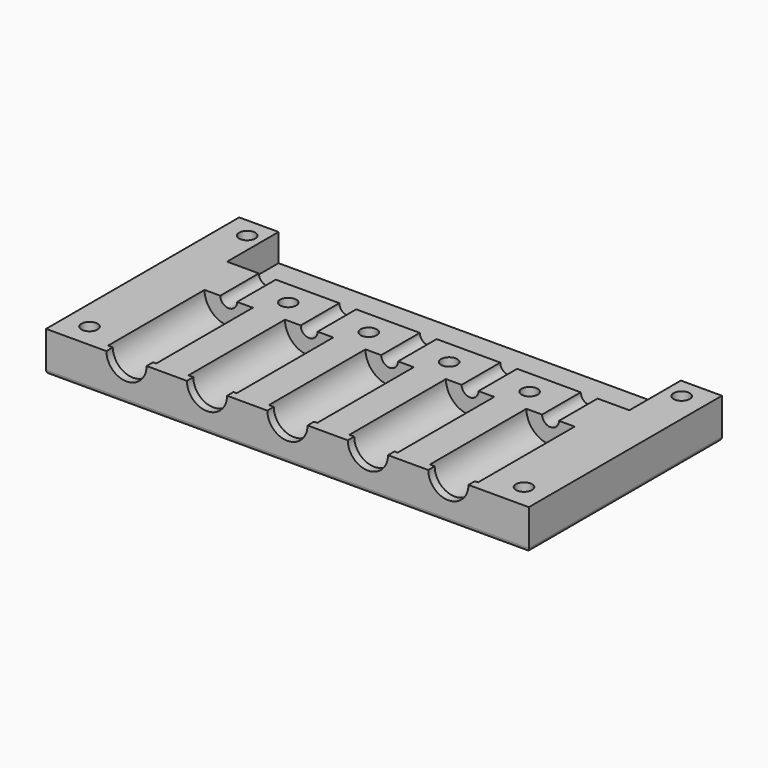
from build123d import *

# Parameters (mm, degrees)
F0_W      = 60
F0_H      = 25
F1_DEPTH  = 5
F2_R      = 2.5
F3_DEPTH  = 10
F5_R      = 3
F6_DEPTH  = 15
F7_R      = 1.05
F8_DEPTH  = 29
F9_W      = 50
F9_H      = 3.4154356362
F10_DEPTH = 3
F11_DEPTH = 5
F12_R     = 0.5
F14_R     = 1
F13_R     = 1
F15_DEPTH = 5.001
F16_R     = 1
F17_DEPTH = 5.001
F18_SIZE  = 1


with BuildPart() as f1:
    # F0 (on Top) → F1 (new body)
    with BuildSketch(Plane.XY):
        with Locations((-2.9453901201, -7.2920476746)):
            Rectangle(F0_W, F0_H)
    extrude(amount=F1_DEPTH)

    # F2 (on face) → F3 (cut)
    with BuildSketch(Plane.XZ.offset(19.7920476746)):
        with Locations((-22.9453901201, 5)):
            Circle(F2_R)
        with Locations((-12.9453901201, 5)):
            Circle(F2_R)
        with Locations((-2.9453901201, 5)):
            Circle(F2_R)
        with Locations((7.0546098799, 5)):
            Circle(F2_R)
        with Locations((17.0546098799, 5)):
            Circle(F2_R)
    extrude(amount=-F3_DEPTH, mode=Mode.SUBTRACT)

    # F5 (on offset) → F6 (cut)
    with BuildSketch(Plane.XZ.offset(18.7920476746)):
        with Locations((-23.0476632714, 5.0127296709)):
            Circle(F5_R)
        with Locations((-13.0476632714, 5.0127296709)):
            Circle(F5_R)
        with Locations((-3.0476632714, 5.0127296709)):
            Circle(F5_R)
        with Locations((6.9523367286, 5.0127296709)):
            Circle(F5_R)
        with Locations((16.9523367286, 5.0127296709)):
            Circle(F5_R)
    extrude(amount=-F6_DEPTH, mode=Mode.SUBTRACT)

    # F7 (on face) → F8 (cut)
    with BuildSketch(Plane.XZ.offset(3.7920476746)):
        with Locations((-23.0476632714, 5.0127296709)):
            Circle(F7_R)
        with Locations((-13.0476632714, 5.0127296709)):
            Circle(F7_R)
        with Locations((-3.0476632714, 5.0127296709)):
            Circle(F7_R)
        with Locations((6.9523367286, 5.0127296709)):
            Circle(F7_R)
        with Locations((16.9523367286, 5.0127296709)):
            Circle(F7_R)
    extrude(amount=-F8_DEPTH, mode=Mode.SUBTRACT)

    # F9 (on face) → F10 (cut)
    with BuildSketch(Plane(origin=(0, 5.2079523254, 0), x_dir=(-1, 0, 0), z_dir=(0, 1, 0))):
        with Locations((3.0476632714, 3.2922821819)):
            Rectangle(F9_W, F9_H)
    extrude(amount=-F10_DEPTH, mode=Mode.SUBTRACT)

    # F11 (add): a face of the model
    f11_faces = [f1.faces().sort_by_distance(p)[0] for p in [
        (-2.8102387692, 5.2079523254, 1.4530193808),
    ]]
    extrude(f11_faces, amount=F11_DEPTH)

    # F12
    f12_edges = [f1.edges().sort_by_distance(p)[0] for p in [
        (27.05461, -4.792048, 0),
        (-2.94539, -19.792048, 0),
        (-32.94539, -4.792048, 0),
    ]]
    fillet(f12_edges, radius=F12_R)

    # F14 (on face) + F13 (on face) → F15 (cut, through all)
    with BuildSketch(Plane(origin=(0, 0, 0), x_dir=(1, 0, 0), z_dir=(0, 0, -1))):
        with Locations((-29.9453901201, -7.7079523254)):
            Circle(F14_R)
        with Locations((24.0546098799, -7.7079523254)):
            Circle(F14_R)
    with BuildSketch(Plane(origin=(0, 0, 0), x_dir=(1, 0, 0), z_dir=(0, 0, -1))):
        with Locations((-29.9453901201, 16.7920476746)):
            Circle(F13_R)
        with Locations((24.0546098799, 16.7920476746)):
            Circle(F13_R)
    extrude(amount=-F15_DEPTH, mode=Mode.SUBTRACT)

    # F16 (on face) → F17 (cut, through all)
    with BuildSketch(Plane.XY.offset(5)):
        with Locations((11.9524138955, -0.7920476746)):
            Circle(F16_R)
        with Locations((1.9524138955, -0.7920476746)):
            Circle(F16_R)
        with Locations((-8.0475861045, -0.7920476746)):
            Circle(F16_R)
        with Locations((-18.0475861045, -0.7920476746)):
            Circle(F16_R)
    extrude(amount=-F17_DEPTH, mode=Mode.SUBTRACT)

    # F18
    f18_edges = [f1.edges().sort_by_distance(p)[0] for p in [
        (23.05461, 7.707952, 0),
        (10.952414, -0.792048, 0),
        (23.05461, -16.792048, 0),
        (0.952414, -0.792048, 0),
        (-9.047586, -0.792048, 0),
        (-19.047586, -0.792048, 0),
        (-30.94539, 7.707952, 0),
        (-30.94539, -16.792048, 0),
    ]]
    chamfer(f18_edges, length=F18_SIZE)


solid = f1.part
